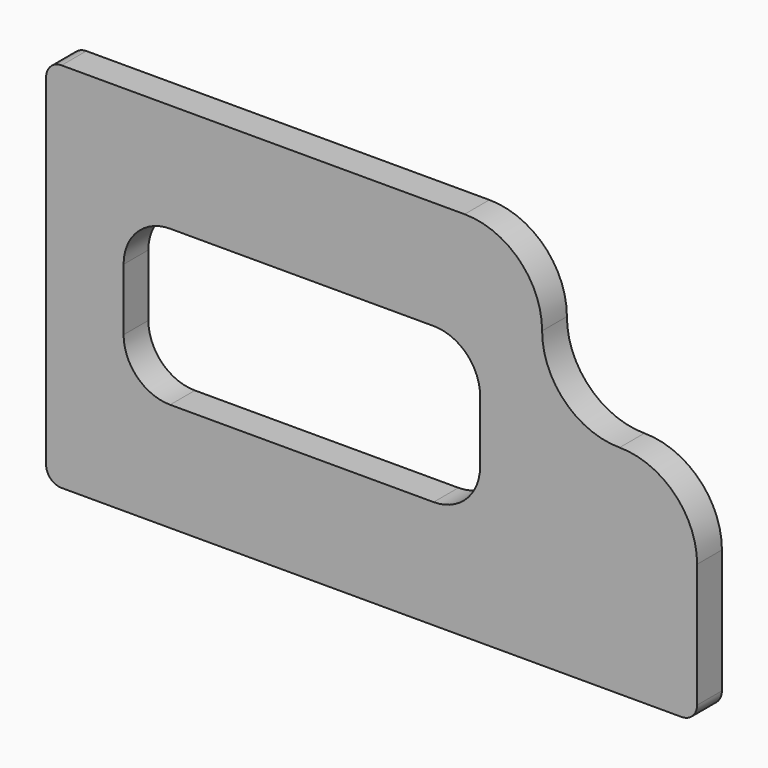
from build123d import *

# Parameters (mm, degrees)
F0_W     = 115
F0_H     = 50
F1_DEPTH = 5
F2_R     = 24.99999
F3_R     = 5
F4_R     = 15


# Not quite as in the source:
# - a fillet or chamfer is up to 0.001 mm smaller than in the source, because OpenCascade refuses the exact size


with BuildPart() as f1:
    # F0 (on Front) → F1 (new body, symmetric)
    with BuildSketch(Plane.XZ):
        Polygon((55, 60), (-105, 60), (-105, -60), (105, -60), (105, 10), (55, 10), align=None)
        with Locations((-22.5, 0)):
            Rectangle(F0_W, F0_H, mode=Mode.SUBTRACT)
    extrude(amount=F1_DEPTH, both=True)

    # F2 (radius 25 in the source; OpenCascade refuses exactly that, so slightly less here)
    f2_edges = [f1.edges().sort_by_distance(p)[0] for p in [
        (55, 0, 10),
        (105, 0, 10),
        (55, 0, 60),
    ]]
    fillet(f2_edges, radius=F2_R)

    # F3
    f3_edges = [f1.edges().sort_by_distance(p)[0] for p in [
        (105, 0, -60),
        (-105, 0, -60),
        (-105, 0, 60),
    ]]
    fillet(f3_edges, radius=F3_R)

    # F4
    f4_edges = [f1.edges().sort_by_distance(p)[0] for p in [
        (-80, 0, -25),
        (35, 0, -25),
        (35, 0, 25),
        (-80, 0, 25),
    ]]
    fillet(f4_edges, radius=F4_R)


solid = f1.part
